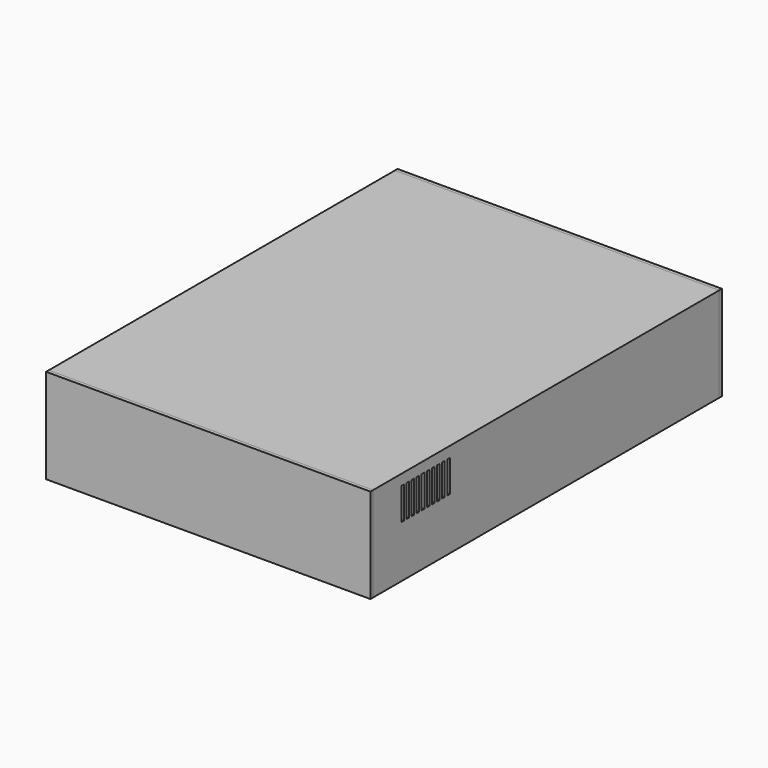
from build123d import *

# Parameters (mm, degrees)
F0_W      = 152.4
F0_H      = 44.45
F1_DEPTH  = 203.2
F2_W      = 149.1996
F2_H      = 41.2496
F3_DEPTH  = 203.201
F7_W      = 152.4
F7_H      = 44.45
F8_DEPTH  = 1.6002
F9_W      = 152.4
F9_H      = 44.45
F10_DEPTH = 1.6002
F11_W     = 1.5
F11_H     = 15
F12_DEPTH = 152.401
F13_W     = 25.4
F13_H     = 25.4
F14_DEPTH = 15
F15_W     = 25.4
F15_H     = 25.4
F16_DEPTH = 1
F17_W     = 25.4
F17_H     = 25.4
F18_DEPTH = 2
F19_W     = 2.54
F19_H     = 25.4
F20_DEPTH = 15
F21_W     = 1.5
F21_H     = 20
F22_DEPTH = 25


# Not quite as in the source:
# - a feature of the source that left no trace in its solid (it failed there, or was rolled back) is left out


with BuildPart() as f1:
    # F0 (on Front) → F1 (new body)
    with BuildSketch(Plane.XZ):
        Rectangle(F0_W, F0_H)
    extrude(amount=-F1_DEPTH)

    # F2 (on face) → F3 (cut, through all)
    with BuildSketch(Plane(origin=(0, 203.2, 0), x_dir=(-1, 0, 0), z_dir=(0, 1, 0))):
        Rectangle(F2_W, F2_H)
    extrude(amount=-F3_DEPTH, mode=Mode.SUBTRACT)

    # F11 (on face) → F12 (cut, through all)
    with BuildSketch(Plane(origin=(-76.2, 0, 0), x_dir=(0, -1, 0), z_dir=(-1, 0, 0))):
        with Locations((-44.25, 9.725)):
            Rectangle(F11_W, F11_H)
        with Locations((-41.25, 9.725)):
            Rectangle(F11_W, F11_H)
        with Locations((-38.25, 9.725)):
            Rectangle(F11_W, F11_H)
        with Locations((-35.25, 9.725)):
            Rectangle(F11_W, F11_H)
        with Locations((-32.25, 9.725)):
            Rectangle(F11_W, F11_H)
        with Locations((-29.25, 9.725)):
            Rectangle(F11_W, F11_H)
        with Locations((-26.25, 9.725)):
            Rectangle(F11_W, F11_H)
        with Locations((-23.25, 9.725)):
            Rectangle(F11_W, F11_H)
        with Locations((-20.25, 9.725)):
            Rectangle(F11_W, F11_H)
        with Locations((-17.25, 9.725)):
            Rectangle(F11_W, F11_H)
    extrude(amount=-F12_DEPTH, mode=Mode.SUBTRACT)


with BuildPart() as f8:
    # F7 (on face) → F8 (new body)
    with BuildSketch(Plane(origin=(0, 203.2, 0), x_dir=(-1, 0, 0), z_dir=(0, 1, 0))):
        Rectangle(F7_W, F7_H)
    extrude(amount=F8_DEPTH)

    # F21 (on face) → F22 (cut)
    with BuildSketch(Plane(origin=(0, 204.8002, 0), x_dir=(-1, 0, 0), z_dir=(0, 1, 0))):
        Rectangle(F21_W, F21_H)
        with Locations((3, 0)):
            Rectangle(F21_W, F21_H)
        with Locations((6, 0)):
            Rectangle(F21_W, F21_H)
        with Locations((9, 0)):
            Rectangle(F21_W, F21_H)
        with Locations((12, 0)):
            Rectangle(F21_W, F21_H)
    extrude(amount=-F22_DEPTH, mode=Mode.SUBTRACT)


with BuildPart() as f10:
    # F9 (on face) → F10 (new body)
    with BuildSketch(Plane.XZ):
        Rectangle(F9_W, F9_H)
    extrude(amount=F10_DEPTH)


with BuildPart() as f14:
    # F13 (on face) → F14 (new body)
    with BuildSketch(Plane.XY.offset(-20.6248)):
        with Locations((0, 75)):
            Rectangle(F13_W, F13_H)
    extrude(amount=F14_DEPTH)


with BuildPart() as f16:
    # F15 (on face) → F16 (new body)
    with BuildSketch(Plane.XY.offset(-5.6248)):
        with Locations((0, 75)):
            Rectangle(F15_W, F15_H)
    extrude(amount=F16_DEPTH)


with BuildPart() as f18:
    # F17 (on face) → F18 (new body)
    with BuildSketch(Plane.XY.offset(-4.6248)):
        with Locations((0, 75)):
            Rectangle(F17_W, F17_H)
    extrude(amount=F18_DEPTH)

    # F19 (on face) → F20 (join)
    with BuildSketch(Plane.XY.offset(-2.6248)):
        with Locations((-11.43, 75)):
            Rectangle(F19_W, F19_H)
        with Locations((-6.35, 75)):
            Rectangle(F19_W, F19_H)
        with Locations((-1.27, 75)):
            Rectangle(F19_W, F19_H)
        with Locations((3.81, 75)):
            Rectangle(F19_W, F19_H)
        with Locations((8.89, 75)):
            Rectangle(F19_W, F19_H)
    extrude(amount=F20_DEPTH)


solid = Compound([f1.part, f8.part, f10.part, f14.part, f16.part, f18.part])
